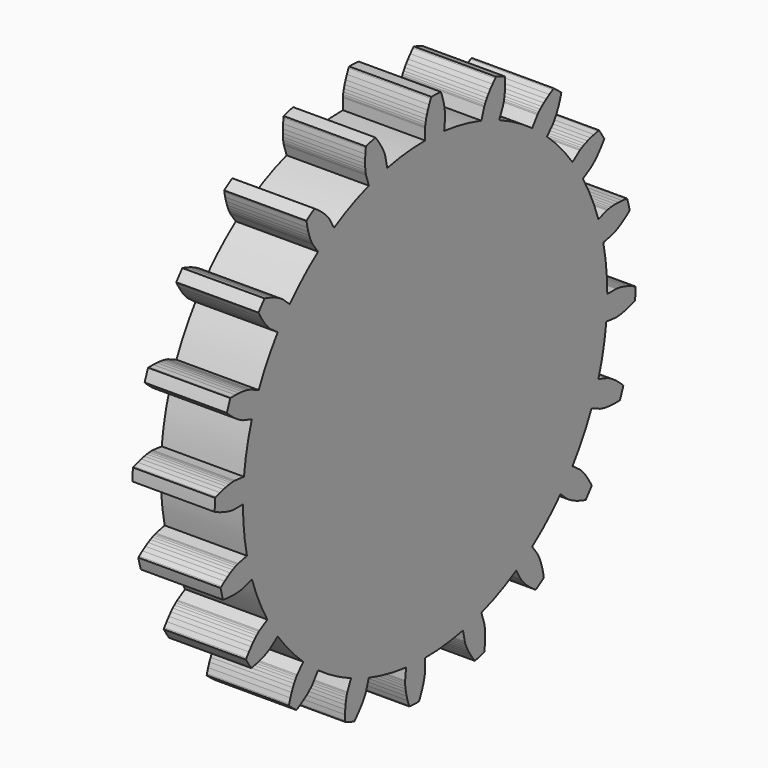
from build123d import *

# Parameters (mm, degrees)
F2_DEPTH = 12.7


# Not quite as in the source:
# - a variable given as a bare number and used for a length is read in inches; the dataset says mm whatever the document's units were


with BuildPart() as f2:
    # F1 (on Right) → F2 (new body)
    with BuildSketch(Plane.YZ):
        with BuildLine():
            ThreePointArc((34.9686031579, -3.6753482932), (35.11303277, -1.8401960714), (35.16122, 0))
            ThreePointArc((35.16122, 0), (34.9686031579, 3.6753482932), (34.3928629819, 7.3104287014))
            ThreePointArc((34.3928629819, 7.3104287014), (33.9631304818, 9.100393385), (33.4403074019, 10.865414523))
            ThreePointArc((33.4403074019, 10.865414523), (32.1213728162, 14.3013565892), (30.4505097481, 17.58061))
            ThreePointArc((30.4505097481, 17.58061), (29.4886803471, 19.1501729308), (28.446024523, 20.6672465686))
            ThreePointArc((28.446024523, 20.6672465686), (26.1298787005, 23.5274484589), (23.5274484589, 26.1298787005))
            ThreePointArc((23.5274484589, 26.1298787005), (22.1276727202, 27.3254001229), (20.6672465686, 28.446024523))
            ThreePointArc((20.6672465686, 28.446024523), (17.58061, 30.4505097481), (14.3013565892, 32.1213728162))
            ThreePointArc((14.3013565892, 32.1213728162), (12.6006543149, 32.8258267638), (10.865414523, 33.4403074019))
            ThreePointArc((10.865414523, 33.4403074019), (7.3104287014, 34.3928629819), (3.6753482932, 34.9686031579))
            ThreePointArc((3.6753482932, 34.9686031579), (1.8401960714, 35.11303277), (0, 35.16122))
            ThreePointArc((0, 35.16122), (-3.6753482932, 34.9686031579), (-7.3104287014, 34.3928629819))
            ThreePointArc((-7.3104287014, 34.3928629819), (-9.100393385, 33.9631304818), (-10.865414523, 33.4403074019))
            ThreePointArc((-10.865414523, 33.4403074019), (-14.3013565892, 32.1213728162), (-17.58061, 30.4505097481))
            ThreePointArc((-17.58061, 30.4505097481), (-19.1501729308, 29.4886803471), (-20.6672465686, 28.446024523))
            ThreePointArc((-20.6672465686, 28.446024523), (-23.5274484589, 26.1298787005), (-26.1298787005, 23.5274484589))
            ThreePointArc((-26.1298787005, 23.5274484589), (-27.3254001229, 22.1276727202), (-28.446024523, 20.6672465686))
            ThreePointArc((-28.446024523, 20.6672465686), (-30.4505097481, 17.58061), (-32.1213728162, 14.3013565892))
            ThreePointArc((-32.1213728162, 14.3013565892), (-32.8258267638, 12.6006543149), (-33.4403074019, 10.865414523))
            ThreePointArc((-33.4403074019, 10.865414523), (-34.3928629819, 7.3104287014), (-34.9686031579, 3.6753482932))
            ThreePointArc((-34.9686031579, 3.6753482932), (-35.11303277, 1.8401960714), (-35.16122, 0))
            ThreePointArc((-35.16122, 0), (-34.9686031579, -3.6753482932), (-34.3928629819, -7.3104287014))
            ThreePointArc((-34.3928629819, -7.3104287014), (-33.9631304818, -9.100393385), (-33.4403074019, -10.865414523))
            ThreePointArc((-33.4403074019, -10.865414523), (-32.1213728162, -14.3013565892), (-30.4505097481, -17.58061))
            ThreePointArc((-30.4505097481, -17.58061), (-29.4886803471, -19.1501729308), (-28.446024523, -20.6672465686))
            ThreePointArc((-28.446024523, -20.6672465686), (-26.1298787005, -23.5274484589), (-23.5274484589, -26.1298787005))
            ThreePointArc((-23.5274484589, -26.1298787005), (-22.1276727202, -27.3254001229), (-20.6672465686, -28.446024523))
            ThreePointArc((-20.6672465686, -28.446024523), (-17.58061, -30.4505097481), (-14.3013565892, -32.1213728162))
            ThreePointArc((-14.3013565892, -32.1213728162), (-12.6006543149, -32.8258267638), (-10.865414523, -33.4403074019))
            ThreePointArc((-10.865414523, -33.4403074019), (-7.3104287014, -34.3928629819), (-3.6753482932, -34.9686031579))
            ThreePointArc((-3.6753482932, -34.9686031579), (-1.8401960714, -35.11303277), (0, -35.16122))
            ThreePointArc((0, -35.16122), (3.6753482932, -34.9686031579), (7.3104287014, -34.3928629819))
            ThreePointArc((7.3104287014, -34.3928629819), (9.100393385, -33.9631304818), (10.865414523, -33.4403074019))
            ThreePointArc((10.865414523, -33.4403074019), (14.3013565892, -32.1213728162), (17.58061, -30.4505097481))
            ThreePointArc((17.58061, -30.4505097481), (19.1501729308, -29.4886803471), (20.6672465686, -28.446024523))
            ThreePointArc((20.6672465686, -28.446024523), (23.5274484589, -26.1298787005), (26.1298787005, -23.5274484589))
            ThreePointArc((26.1298787005, -23.5274484589), (27.3254001229, -22.1276727202), (28.446024523, -20.6672465686))
            ThreePointArc((28.446024523, -20.6672465686), (30.4505097481, -17.58061), (32.1213728162, -14.3013565892))
            ThreePointArc((32.1213728162, -14.3013565892), (32.8258267638, -12.6006543149), (33.4403074019, -10.865414523))
            ThreePointArc((33.4403074019, -10.865414523), (34.3928629819, -7.3104287014), (34.9686031579, -3.6753482932))
        make_face()
        with BuildLine():
            Line((-35.0810749527, -11.3985322171), (-33.4403074019, -10.865414523))
            ThreePointArc((-33.4403074019, -10.865414523), (-33.9631304818, -9.100393385), (-34.3928629819, -7.3104287014))
            Line((-34.3928629819, -7.3104287014), (-36.0803682097, -7.6691190104))
            Line((-36.0803682097, -7.6691190104), (-36.125121025, -7.6802023647))
            Line((-36.125121025, -7.6802023647), (-36.2577654905, -7.7193835081))
            Line((-36.2577654905, -7.7193835081), (-36.4753836489, -7.7954109725))
            Line((-36.4753836489, -7.7954109725), (-36.7744062464, -7.9168008706))
            Line((-36.7744062464, -7.9168008706), (-37.1506292157, -8.0917938492))
            Line((-37.1506292157, -8.0917938492), (-37.5992328238, -8.3283131361))
            Line((-37.5992328238, -8.3283131361), (-38.1148034149, -8.633923839))
            Line((-38.1148034149, -8.633923839), (-38.6913576712, -9.0157936503))
            Line((-38.6913576712, -9.0157936503), (-39.3223693016, -9.4806551065))
            Line((-39.3223693016, -9.4806551065), (-39.4863231421, -9.6145662784))
            ThreePointArc((-39.4863231421, -9.6145662784), (-39.2552255804, -10.518405993), (-39.0034420822, -11.4167029276))
            Line((-39.0034420822, -11.4167029276), (-38.7944983054, -11.450696484))
            Line((-38.7944983054, -11.450696484), (-38.0155954753, -11.5377724992))
            Line((-38.0155954753, -11.5377724992), (-37.3253499371, -11.5802043285))
            Line((-37.3253499371, -11.5802043285), (-36.7260473563, -11.5870856653))
            Line((-36.7260473563, -11.5870856653), (-36.219285592, -11.5676155722))
            Line((-36.219285592, -11.5676155722), (-35.8059704538, -11.5310524525))
            Line((-35.8059704538, -11.5310524525), (-35.486314339, -11.4866678893))
            Line((-35.486314339, -11.4866678893), (-35.2598377532, -11.4437005257))
            Line((-35.2598377532, -11.4437005257), (-35.1253737048, -11.4113101584))
            Line((-35.1253737048, -11.4113101584), (-35.0810749527, -11.3985322171))
        make_face()
        with BuildLine():
            Line((-29.8417447663, -21.6812966826), (-28.446024523, -20.6672465686))
            ThreePointArc((-28.446024523, -20.6672465686), (-29.4886803471, -19.1501729308), (-30.4505097481, -17.58061))
            Line((-30.4505097481, -17.58061), (-31.94458119, -18.4432125492))
            Line((-31.94458119, -18.4432125492), (-31.9837187018, -18.467582826))
            Line((-31.9837187018, -18.467582826), (-32.0977634459, -18.5458357018))
            Line((-32.0977634459, -18.5458357018), (-32.281236835, -18.6853898264))
            Line((-32.281236835, -18.6853898264), (-32.5281126834, -18.8932415444))
            Line((-32.5281126834, -18.8932415444), (-32.8318461857, -19.1759290482))
            Line((-32.8318461857, -19.1759290482), (-33.1854050912, -19.5394983959))
            Line((-33.1854050912, -19.5394983959), (-33.5813029607, -19.9894715208))
            Line((-33.5813029607, -19.9894715208), (-34.0116343818, -20.5308163565))
            Line((-34.0116343818, -20.5308163565), (-34.4681120147, -21.1679191911))
            Line((-34.4681120147, -21.1679191911), (-34.5826605552, -21.3459408067))
            ThreePointArc((-34.5826605552, -21.3459408067), (-34.0835718813, -22.134130383), (-33.5665225259, -22.9106561564))
            Line((-33.5665225259, -22.9106561564), (-33.3573005988, -22.8784187719))
            Line((-33.3573005988, -22.8784187719), (-32.5896120182, -22.7205387721))
            Line((-32.5896120182, -22.7205387721), (-31.9200373448, -22.5475962382))
            Line((-31.9200373448, -22.5475962382), (-31.3479402701, -22.3689460962))
            Line((-31.3479402701, -22.3689460962), (-30.8719977816, -22.19383094))
            Line((-30.8719977816, -22.19383094), (-30.4902103515, -22.031335945))
            Line((-30.4902103515, -22.031335945), (-30.1999149048, -21.8903445451))
            Line((-30.1999149048, -21.8903445451), (-29.9978005178, -21.7794950401))
            Line((-29.9978005178, -21.7794950401), (-29.8799267822, -21.7071382942))
            Line((-29.8799267822, -21.7071382942), (-29.8417447663, -21.6812966826))
        make_face()
        with BuildLine():
            Line((-21.6812966826, -29.8417447663), (-20.6672465686, -28.446024523))
            ThreePointArc((-20.6672465686, -28.446024523), (-22.1276727202, -27.3254001229), (-23.5274484589, -26.1298787005))
            Line((-23.5274484589, -26.1298787005), (-24.6818359925, -27.4119559422))
            Line((-24.6818359925, -27.4119559422), (-24.7115271484, -27.4472276091))
            Line((-24.7115271484, -27.4472276091), (-24.795808677, -27.5568922805))
            Line((-24.795808677, -27.5568922805), (-24.9271776431, -27.7463125354))
            Line((-24.9271776431, -27.7463125354), (-25.0977408143, -28.0202800989))
            Line((-25.0977408143, -28.0202800989), (-25.2992532981, -28.3829907054))
            Line((-25.2992532981, -28.3829907054), (-25.523158692, -28.8380214129))
            Line((-25.523158692, -28.8380214129), (-25.7606305979, -29.3883104552))
            Line((-25.7606305979, -29.3883104552), (-26.0026153461, -30.0361397112))
            Line((-26.0026153461, -30.0361397112), (-26.2398757704, -30.7831198597))
            Line((-26.2398757704, -30.7831198597), (-26.2938062017, -30.9878259229))
            ThreePointArc((-26.2938062017, -30.9878259229), (-25.5755806923, -31.5832118736), (-24.843877873, -32.1619547327))
            Line((-24.843877873, -32.1619547327), (-24.6548578956, -32.066642027))
            Line((-24.6548578956, -32.066642027), (-23.9735302715, -31.6792604066))
            Line((-23.9735302715, -31.6792604066), (-23.3901690973, -31.3078723298))
            Line((-23.3901690973, -31.3078723298), (-22.9012783763, -30.9611782295))
            Line((-22.9012783763, -30.9611782295), (-22.5027437305, -30.6475595019))
            Line((-22.5027437305, -30.6475595019), (-22.1898560222, -30.3750387739))
            Line((-22.1898560222, -30.3750387739), (-21.9573373846, -30.1512417578))
            Line((-21.9573373846, -30.1512417578), (-21.7993695606, -29.9833608334))
            Line((-21.7993695606, -29.9833608334), (-21.7096244405, -29.8781204912))
            Line((-21.7096244405, -29.8781204912), (-21.6812966826, -29.8417447663))
        make_face()
        with BuildLine():
            Line((-11.3985322171, -35.0810749527), (-10.865414523, -33.4403074019))
            ThreePointArc((-10.865414523, -33.4403074019), (-12.6006543149, -32.8258267638), (-14.3013565892, -32.1213728162))
            Line((-14.3013565892, -32.1213728162), (-15.0030607196, -33.6974260973))
            Line((-15.0030607196, -33.6974260973), (-15.0203991425, -33.7401465177))
            Line((-15.0203991425, -33.7401465177), (-15.0666673922, -33.8704882427))
            Line((-15.0666673922, -33.8704882427), (-15.1330726256, -34.0912328535))
            Line((-15.1330726256, -34.0912328535), (-15.210627208, -34.4044984085))
            Line((-15.210627208, -34.4044984085), (-15.2901932274, -34.8117274764))
            Line((-15.2901932274, -34.8117274764), (-15.3625276897, -35.3136779678))
            Line((-15.3625276897, -35.3136779678), (-15.4183282274, -35.9104168019))
            Line((-15.4183282274, -35.9104168019), (-15.4482791495, -36.6013164368))
            Line((-15.4482791495, -36.6013164368), (-15.4430976617, -37.3850542778))
            Line((-15.4430976617, -37.3850542778), (-15.4311308974, -37.5964067329))
            ThreePointArc((-15.4311308974, -37.5964067329), (-14.5640734695, -37.9407085328), (-13.6893413564, -38.2650170943))
            Line((-13.6893413564, -38.2650170943), (-13.539025921, -38.1159589391))
            Line((-13.539025921, -38.1159589391), (-13.0107523484, -37.5369953102))
            Line((-13.0107523484, -37.5369953102), (-12.5707081296, -37.0035157429))
            Line((-12.5707081296, -37.0035157429), (-12.2128797925, -36.5227145185))
            Line((-12.2128797925, -36.5227145185), (-11.9307643372, -36.1012914056))
            Line((-11.9307643372, -36.1012914056), (-11.7174039796, -35.7454211722))
            Line((-11.7174039796, -35.7454211722), (-11.5654226955, -35.4607253513))
            Line((-11.5654226955, -35.4607253513), (-11.4670644258, -35.2522463619))
            Line((-11.4670644258, -35.2522463619), (-11.4142327987, -35.1244240814))
            Line((-11.4142327987, -35.1244240814), (-11.3985322171, -35.0810749527))
        make_face()
        with BuildLine():
            Line((0, -36.8864250984), (0, -35.16122))
            ThreePointArc((0, -35.16122), (-1.8401960714, -35.11303277), (-3.6753482932, -34.9686031579))
            Line((-3.6753482932, -34.9686031579), (-3.855681331, -36.6843574022))
            Line((-3.855681331, -36.6843574022), (-3.8589698151, -36.7303448037))
            Line((-3.8589698151, -36.7303448037), (-3.8626957275, -36.8686048261))
            Line((-3.8626957275, -36.8686048261), (-3.8576370213, -37.0990657723))
            Line((-3.8576370213, -37.0990657723), (-3.834591432, -37.4209647036))
            Line((-3.834591432, -37.4209647036), (-3.7844225105, -37.8328498145))
            Line((-3.7844225105, -37.8328498145), (-3.6981054401, -38.3325856783))
            Line((-3.6981054401, -38.3325856783), (-3.5667724642, -38.9173613495))
            Line((-3.5667724642, -38.9173613495), (-3.3817577552, -39.5837012932))
            Line((-3.3817577552, -39.5837012932), (-3.1346415555, -40.3274791062))
            Line((-3.1346415555, -40.3274791062), (-3.0579489859, -40.5247893023))
            ThreePointArc((-3.0579489859, -40.5247893023), (-2.1269332617, -40.5843042924), (-1.1947967286, -40.6224329746))
            Line((-1.1947967286, -40.6224329746), (-1.0978997574, -40.4342202208))
            Line((-1.0978997574, -40.4342202208), (-0.7743913343, -39.7203475771))
            Line((-0.7743913343, -39.7203475771), (-0.5207386649, -39.0769972165))
            Line((-0.5207386649, -39.0769972165), (-0.3289994424, -38.5091530418))
            Line((-0.3289994424, -38.5091530418), (-0.1909186041, -38.0211773741))
            Line((-0.1909186041, -38.0211773741), (-0.0979707956, -37.6167926932))
            Line((-0.0979707956, -37.6167926932), (-0.0414038518, -37.2990660779))
            Line((-0.0414038518, -37.2990660779), (-0.0122831292, -37.0703963997))
            Line((-0.0122831292, -37.0703963997), (-0.0015365229, -36.9325043163))
            Line((-0.0015365229, -36.9325043163), (0, -36.8864250984))
        make_face()
        with BuildLine():
            Line((11.3985322171, -35.0810749527), (10.865414523, -33.4403074019))
            ThreePointArc((10.865414523, -33.4403074019), (9.100393385, -33.9631304818), (7.3104287014, -34.3928629819))
            Line((7.3104287014, -34.3928629819), (7.6691190104, -36.0803682097))
            Line((7.6691190104, -36.0803682097), (7.6802023647, -36.125121025))
            Line((7.6802023647, -36.125121025), (7.7193835081, -36.2577654905))
            Line((7.7193835081, -36.2577654905), (7.7954109725, -36.4753836489))
            Line((7.7954109725, -36.4753836489), (7.9168008706, -36.7744062464))
            Line((7.9168008706, -36.7744062464), (8.0917938492, -37.1506292157))
            Line((8.0917938492, -37.1506292157), (8.3283131361, -37.5992328238))
            Line((8.3283131361, -37.5992328238), (8.633923839, -38.1148034149))
            Line((8.633923839, -38.1148034149), (9.0157936503, -38.6913576712))
            Line((9.0157936503, -38.6913576712), (9.4806551065, -39.3223693016))
            Line((9.4806551065, -39.3223693016), (9.6145662784, -39.4863231421))
            ThreePointArc((9.6145662784, -39.4863231421), (10.518405993, -39.2552255804), (11.4167029276, -39.0034420822))
            Line((11.4167029276, -39.0034420822), (11.450696484, -38.7944983054))
            Line((11.450696484, -38.7944983054), (11.5377724992, -38.0155954753))
            Line((11.5377724992, -38.0155954753), (11.5802043285, -37.3253499371))
            Line((11.5802043285, -37.3253499371), (11.5870856653, -36.7260473563))
            Line((11.5870856653, -36.7260473563), (11.5676155722, -36.219285592))
            Line((11.5676155722, -36.219285592), (11.5310524525, -35.8059704538))
            Line((11.5310524525, -35.8059704538), (11.4866678893, -35.486314339))
            Line((11.4866678893, -35.486314339), (11.4437005257, -35.2598377532))
            Line((11.4437005257, -35.2598377532), (11.4113101584, -35.1253737048))
            Line((11.4113101584, -35.1253737048), (11.3985322171, -35.0810749527))
        make_face()
        with BuildLine():
            Line((21.6812966826, -29.8417447663), (20.6672465686, -28.446024523))
            ThreePointArc((20.6672465686, -28.446024523), (19.1501729308, -29.4886803471), (17.58061, -30.4505097481))
            Line((17.58061, -30.4505097481), (18.4432125492, -31.94458119))
            Line((18.4432125492, -31.94458119), (18.467582826, -31.9837187018))
            Line((18.467582826, -31.9837187018), (18.5458357018, -32.0977634459))
            Line((18.5458357018, -32.0977634459), (18.6853898264, -32.281236835))
            Line((18.6853898264, -32.281236835), (18.8932415444, -32.5281126834))
            Line((18.8932415444, -32.5281126834), (19.1759290482, -32.8318461857))
            Line((19.1759290482, -32.8318461857), (19.5394983959, -33.1854050912))
            Line((19.5394983959, -33.1854050912), (19.9894715208, -33.5813029607))
            Line((19.9894715208, -33.5813029607), (20.5308163565, -34.0116343818))
            Line((20.5308163565, -34.0116343818), (21.1679191911, -34.4681120147))
            Line((21.1679191911, -34.4681120147), (21.3459408067, -34.5826605552))
            ThreePointArc((21.3459408067, -34.5826605552), (22.134130383, -34.0835718813), (22.9106561564, -33.5665225259))
            Line((22.9106561564, -33.5665225259), (22.8784187719, -33.3573005988))
            Line((22.8784187719, -33.3573005988), (22.7205387721, -32.5896120182))
            Line((22.7205387721, -32.5896120182), (22.5475962382, -31.9200373448))
            Line((22.5475962382, -31.9200373448), (22.3689460962, -31.3479402701))
            Line((22.3689460962, -31.3479402701), (22.19383094, -30.8719977816))
            Line((22.19383094, -30.8719977816), (22.031335945, -30.4902103515))
            Line((22.031335945, -30.4902103515), (21.8903445451, -30.1999149048))
            Line((21.8903445451, -30.1999149048), (21.7794950401, -29.9978005178))
            Line((21.7794950401, -29.9978005178), (21.7071382942, -29.8799267822))
            Line((21.7071382942, -29.8799267822), (21.6812966826, -29.8417447663))
        make_face()
        with BuildLine():
            Line((29.8417447663, -21.6812966826), (28.446024523, -20.6672465686))
            ThreePointArc((28.446024523, -20.6672465686), (27.3254001229, -22.1276727202), (26.1298787005, -23.5274484589))
            Line((26.1298787005, -23.5274484589), (27.4119559422, -24.6818359925))
            Line((27.4119559422, -24.6818359925), (27.4472276091, -24.7115271484))
            Line((27.4472276091, -24.7115271484), (27.5568922805, -24.795808677))
            Line((27.5568922805, -24.795808677), (27.7463125354, -24.9271776431))
            Line((27.7463125354, -24.9271776431), (28.0202800989, -25.0977408143))
            Line((28.0202800989, -25.0977408143), (28.3829907054, -25.2992532981))
            Line((28.3829907054, -25.2992532981), (28.8380214129, -25.523158692))
            Line((28.8380214129, -25.523158692), (29.3883104552, -25.7606305979))
            Line((29.3883104552, -25.7606305979), (30.0361397112, -26.0026153461))
            Line((30.0361397112, -26.0026153461), (30.7831198597, -26.2398757704))
            Line((30.7831198597, -26.2398757704), (30.9878259229, -26.2938062017))
            ThreePointArc((30.9878259229, -26.2938062017), (31.5832118736, -25.5755806923), (32.1619547327, -24.843877873))
            Line((32.1619547327, -24.843877873), (32.066642027, -24.6548578956))
            Line((32.066642027, -24.6548578956), (31.6792604066, -23.9735302715))
            Line((31.6792604066, -23.9735302715), (31.3078723298, -23.3901690973))
            Line((31.3078723298, -23.3901690973), (30.9611782295, -22.9012783763))
            Line((30.9611782295, -22.9012783763), (30.6475595019, -22.5027437305))
            Line((30.6475595019, -22.5027437305), (30.3750387739, -22.1898560222))
            Line((30.3750387739, -22.1898560222), (30.1512417578, -21.9573373846))
            Line((30.1512417578, -21.9573373846), (29.9833608334, -21.7993695606))
            Line((29.9833608334, -21.7993695606), (29.8781204912, -21.7096244405))
            Line((29.8781204912, -21.7096244405), (29.8417447663, -21.6812966826))
        make_face()
        with BuildLine():
            Line((35.0810749527, -11.3985322171), (33.4403074019, -10.865414523))
            ThreePointArc((33.4403074019, -10.865414523), (32.8258267638, -12.6006543149), (32.1213728162, -14.3013565892))
            Line((32.1213728162, -14.3013565892), (33.6974260973, -15.0030607196))
            Line((33.6974260973, -15.0030607196), (33.7401465177, -15.0203991425))
            Line((33.7401465177, -15.0203991425), (33.8704882427, -15.0666673922))
            Line((33.8704882427, -15.0666673922), (34.0912328535, -15.1330726256))
            Line((34.0912328535, -15.1330726256), (34.4044984085, -15.210627208))
            Line((34.4044984085, -15.210627208), (34.8117274764, -15.2901932274))
            Line((34.8117274764, -15.2901932274), (35.3136779678, -15.3625276897))
            Line((35.3136779678, -15.3625276897), (35.9104168019, -15.4183282274))
            Line((35.9104168019, -15.4183282274), (36.6013164368, -15.4482791495))
            Line((36.6013164368, -15.4482791495), (37.3850542778, -15.4430976617))
            Line((37.3850542778, -15.4430976617), (37.5964067329, -15.4311308974))
            ThreePointArc((37.5964067329, -15.4311308974), (37.9407085328, -14.5640734695), (38.2650170943, -13.6893413564))
            Line((38.2650170943, -13.6893413564), (38.1159589391, -13.539025921))
            Line((38.1159589391, -13.539025921), (37.5369953102, -13.0107523484))
            Line((37.5369953102, -13.0107523484), (37.0035157429, -12.5707081296))
            Line((37.0035157429, -12.5707081296), (36.5227145185, -12.2128797925))
            Line((36.5227145185, -12.2128797925), (36.1012914056, -11.9307643372))
            Line((36.1012914056, -11.9307643372), (35.7454211722, -11.7174039796))
            Line((35.7454211722, -11.7174039796), (35.4607253513, -11.5654226955))
            Line((35.4607253513, -11.5654226955), (35.2522463619, -11.4670644258))
            Line((35.2522463619, -11.4670644258), (35.1244240814, -11.4142327987))
            Line((35.1244240814, -11.4142327987), (35.0810749527, -11.3985322171))
        make_face()
        with BuildLine():
            Line((36.8864250984, 0), (35.16122, 0))
            ThreePointArc((35.16122, 0), (35.11303277, -1.8401960714), (34.9686031579, -3.6753482932))
            Line((34.9686031579, -3.6753482932), (36.6843574022, -3.855681331))
            Line((36.6843574022, -3.855681331), (36.7303448037, -3.8589698151))
            Line((36.7303448037, -3.8589698151), (36.8686048261, -3.8626957275))
            Line((36.8686048261, -3.8626957275), (37.0990657723, -3.8576370213))
            Line((37.0990657723, -3.8576370213), (37.4209647036, -3.834591432))
            Line((37.4209647036, -3.834591432), (37.8328498145, -3.7844225105))
            Line((37.8328498145, -3.7844225105), (38.3325856783, -3.6981054401))
            Line((38.3325856783, -3.6981054401), (38.9173613495, -3.5667724642))
            Line((38.9173613495, -3.5667724642), (39.5837012932, -3.3817577552))
            Line((39.5837012932, -3.3817577552), (40.3274791062, -3.1346415555))
            Line((40.3274791062, -3.1346415555), (40.5247893023, -3.0579489859))
            ThreePointArc((40.5247893023, -3.0579489859), (40.5843042924, -2.1269332617), (40.6224329746, -1.1947967286))
            Line((40.6224329746, -1.1947967286), (40.4342202208, -1.0978997574))
            Line((40.4342202208, -1.0978997574), (39.7203475771, -0.7743913343))
            Line((39.7203475771, -0.7743913343), (39.0769972165, -0.5207386649))
            Line((39.0769972165, -0.5207386649), (38.5091530418, -0.3289994424))
            Line((38.5091530418, -0.3289994424), (38.0211773741, -0.1909186041))
            Line((38.0211773741, -0.1909186041), (37.6167926932, -0.0979707956))
            Line((37.6167926932, -0.0979707956), (37.2990660779, -0.0414038518))
            Line((37.2990660779, -0.0414038518), (37.0703963997, -0.0122831292))
            Line((37.0703963997, -0.0122831292), (36.9325043163, -0.0015365229))
            Line((36.9325043163, -0.0015365229), (36.8864250984, 0))
        make_face()
        with BuildLine():
            ThreePointArc((33.4403074019, 10.865414523), (33.9631304818, 9.100393385), (34.3928629819, 7.3104287014))
            Line((34.3928629819, 7.3104287014), (36.0803682097, 7.6691190104))
            Line((36.0803682097, 7.6691190104), (36.125121025, 7.6802023647))
            Line((36.125121025, 7.6802023647), (36.2577654905, 7.7193835081))
            Line((36.2577654905, 7.7193835081), (36.4753836489, 7.7954109725))
            Line((36.4753836489, 7.7954109725), (36.7744062464, 7.9168008706))
            Line((36.7744062464, 7.9168008706), (37.1506292157, 8.0917938492))
            Line((37.1506292157, 8.0917938492), (37.5992328238, 8.3283131361))
            Line((37.5992328238, 8.3283131361), (38.1148034149, 8.633923839))
            Line((38.1148034149, 8.633923839), (38.6913576712, 9.0157936503))
            Line((38.6913576712, 9.0157936503), (39.3223693016, 9.4806551065))
            Line((39.3223693016, 9.4806551065), (39.4863231421, 9.6145662784))
            ThreePointArc((39.4863231421, 9.6145662784), (39.2552255804, 10.518405993), (39.0034420822, 11.4167029276))
            Line((39.0034420822, 11.4167029276), (38.7944983054, 11.450696484))
            Line((38.7944983054, 11.450696484), (38.0155954753, 11.5377724992))
            Line((38.0155954753, 11.5377724992), (37.3253499371, 11.5802043285))
            Line((37.3253499371, 11.5802043285), (36.7260473563, 11.5870856653))
            Line((36.7260473563, 11.5870856653), (36.219285592, 11.5676155722))
            Line((36.219285592, 11.5676155722), (35.8059704538, 11.5310524525))
            Line((35.8059704538, 11.5310524525), (35.486314339, 11.4866678893))
            Line((35.486314339, 11.4866678893), (35.2598377532, 11.4437005257))
            Line((35.2598377532, 11.4437005257), (35.1253737048, 11.4113101584))
            Line((35.1253737048, 11.4113101584), (35.0810749527, 11.3985322171))
            Line((35.0810749527, 11.3985322171), (33.4403074019, 10.865414523))
        make_face()
        with BuildLine():
            ThreePointArc((28.446024523, 20.6672465686), (29.4886803471, 19.1501729308), (30.4505097481, 17.58061))
            Line((30.4505097481, 17.58061), (31.94458119, 18.4432125492))
            Line((31.94458119, 18.4432125492), (31.9837187018, 18.467582826))
            Line((31.9837187018, 18.467582826), (32.0977634459, 18.5458357018))
            Line((32.0977634459, 18.5458357018), (32.281236835, 18.6853898264))
            Line((32.281236835, 18.6853898264), (32.5281126834, 18.8932415444))
            Line((32.5281126834, 18.8932415444), (32.8318461857, 19.1759290482))
            Line((32.8318461857, 19.1759290482), (33.1854050912, 19.5394983959))
            Line((33.1854050912, 19.5394983959), (33.5813029607, 19.9894715208))
            Line((33.5813029607, 19.9894715208), (34.0116343818, 20.5308163565))
            Line((34.0116343818, 20.5308163565), (34.4681120147, 21.1679191911))
            Line((34.4681120147, 21.1679191911), (34.5826605552, 21.3459408067))
            ThreePointArc((34.5826605552, 21.3459408067), (34.0835718813, 22.134130383), (33.5665225259, 22.9106561564))
            Line((33.5665225259, 22.9106561564), (33.3573005988, 22.8784187719))
            Line((33.3573005988, 22.8784187719), (32.5896120182, 22.7205387721))
            Line((32.5896120182, 22.7205387721), (31.9200373448, 22.5475962382))
            Line((31.9200373448, 22.5475962382), (31.3479402701, 22.3689460962))
            Line((31.3479402701, 22.3689460962), (30.8719977816, 22.19383094))
            Line((30.8719977816, 22.19383094), (30.4902103515, 22.031335945))
            Line((30.4902103515, 22.031335945), (30.1999149048, 21.8903445451))
            Line((30.1999149048, 21.8903445451), (29.9978005178, 21.7794950401))
            Line((29.9978005178, 21.7794950401), (29.8799267822, 21.7071382942))
            Line((29.8799267822, 21.7071382942), (29.8417447663, 21.6812966826))
            Line((29.8417447663, 21.6812966826), (28.446024523, 20.6672465686))
        make_face()
        with BuildLine():
            ThreePointArc((20.6672465686, 28.446024523), (22.1276727202, 27.3254001229), (23.5274484589, 26.1298787005))
            Line((23.5274484589, 26.1298787005), (24.6818359925, 27.4119559422))
            Line((24.6818359925, 27.4119559422), (24.7115271484, 27.4472276091))
            Line((24.7115271484, 27.4472276091), (24.795808677, 27.5568922805))
            Line((24.795808677, 27.5568922805), (24.9271776431, 27.7463125354))
            Line((24.9271776431, 27.7463125354), (25.0977408143, 28.0202800989))
            Line((25.0977408143, 28.0202800989), (25.2992532981, 28.3829907054))
            Line((25.2992532981, 28.3829907054), (25.523158692, 28.8380214129))
            Line((25.523158692, 28.8380214129), (25.7606305979, 29.3883104552))
            Line((25.7606305979, 29.3883104552), (26.0026153461, 30.0361397112))
            Line((26.0026153461, 30.0361397112), (26.2398757704, 30.7831198597))
            Line((26.2398757704, 30.7831198597), (26.2938062017, 30.9878259229))
            ThreePointArc((26.2938062017, 30.9878259229), (25.5755806923, 31.5832118736), (24.843877873, 32.1619547327))
            Line((24.843877873, 32.1619547327), (24.6548578956, 32.066642027))
            Line((24.6548578956, 32.066642027), (23.9735302715, 31.6792604066))
            Line((23.9735302715, 31.6792604066), (23.3901690973, 31.3078723298))
            Line((23.3901690973, 31.3078723298), (22.9012783763, 30.9611782295))
            Line((22.9012783763, 30.9611782295), (22.5027437305, 30.6475595019))
            Line((22.5027437305, 30.6475595019), (22.1898560222, 30.3750387739))
            Line((22.1898560222, 30.3750387739), (21.9573373846, 30.1512417578))
            Line((21.9573373846, 30.1512417578), (21.7993695606, 29.9833608334))
            Line((21.7993695606, 29.9833608334), (21.7096244405, 29.8781204912))
            Line((21.7096244405, 29.8781204912), (21.6812966826, 29.8417447663))
            Line((21.6812966826, 29.8417447663), (20.6672465686, 28.446024523))
        make_face()
        with BuildLine():
            ThreePointArc((10.865414523, 33.4403074019), (12.6006543149, 32.8258267638), (14.3013565892, 32.1213728162))
            Line((14.3013565892, 32.1213728162), (15.0030607196, 33.6974260973))
            Line((15.0030607196, 33.6974260973), (15.0203991425, 33.7401465177))
            Line((15.0203991425, 33.7401465177), (15.0666673922, 33.8704882427))
            Line((15.0666673922, 33.8704882427), (15.1330726256, 34.0912328535))
            Line((15.1330726256, 34.0912328535), (15.210627208, 34.4044984085))
            Line((15.210627208, 34.4044984085), (15.2901932274, 34.8117274764))
            Line((15.2901932274, 34.8117274764), (15.3625276897, 35.3136779678))
            Line((15.3625276897, 35.3136779678), (15.4183282274, 35.9104168019))
            Line((15.4183282274, 35.9104168019), (15.4482791495, 36.6013164368))
            Line((15.4482791495, 36.6013164368), (15.4430976617, 37.3850542778))
            Line((15.4430976617, 37.3850542778), (15.4311308974, 37.5964067329))
            ThreePointArc((15.4311308974, 37.5964067329), (14.5640734695, 37.9407085328), (13.6893413564, 38.2650170943))
            Line((13.6893413564, 38.2650170943), (13.539025921, 38.1159589391))
            Line((13.539025921, 38.1159589391), (13.0107523484, 37.5369953102))
            Line((13.0107523484, 37.5369953102), (12.5707081296, 37.0035157429))
            Line((12.5707081296, 37.0035157429), (12.2128797925, 36.5227145185))
            Line((12.2128797925, 36.5227145185), (11.9307643372, 36.1012914056))
            Line((11.9307643372, 36.1012914056), (11.7174039796, 35.7454211722))
            Line((11.7174039796, 35.7454211722), (11.5654226955, 35.4607253513))
            Line((11.5654226955, 35.4607253513), (11.4670644258, 35.2522463619))
            Line((11.4670644258, 35.2522463619), (11.4142327987, 35.1244240814))
            Line((11.4142327987, 35.1244240814), (11.3985322171, 35.0810749527))
            Line((11.3985322171, 35.0810749527), (10.865414523, 33.4403074019))
        make_face()
        with BuildLine():
            ThreePointArc((0, 35.16122), (1.8401960714, 35.11303277), (3.6753482932, 34.9686031579))
            Line((3.6753482932, 34.9686031579), (3.855681331, 36.6843574022))
            Line((3.855681331, 36.6843574022), (3.8589698151, 36.7303448037))
            Line((3.8589698151, 36.7303448037), (3.8626957275, 36.8686048261))
            Line((3.8626957275, 36.8686048261), (3.8576370213, 37.0990657723))
            Line((3.8576370213, 37.0990657723), (3.834591432, 37.4209647036))
            Line((3.834591432, 37.4209647036), (3.7844225105, 37.8328498145))
            Line((3.7844225105, 37.8328498145), (3.6981054401, 38.3325856783))
            Line((3.6981054401, 38.3325856783), (3.5667724642, 38.9173613495))
            Line((3.5667724642, 38.9173613495), (3.3817577552, 39.5837012932))
            Line((3.3817577552, 39.5837012932), (3.1346415555, 40.3274791062))
            Line((3.1346415555, 40.3274791062), (3.0579489859, 40.5247893023))
            ThreePointArc((3.0579489859, 40.5247893023), (2.1269332617, 40.5843042924), (1.1947967286, 40.6224329746))
            Line((1.1947967286, 40.6224329746), (1.0978997574, 40.4342202208))
            Line((1.0978997574, 40.4342202208), (0.7743913343, 39.7203475771))
            Line((0.7743913343, 39.7203475771), (0.5207386649, 39.0769972165))
            Line((0.5207386649, 39.0769972165), (0.3289994424, 38.5091530418))
            Line((0.3289994424, 38.5091530418), (0.1909186041, 38.0211773741))
            Line((0.1909186041, 38.0211773741), (0.0979707956, 37.6167926932))
            Line((0.0979707956, 37.6167926932), (0.0414038518, 37.2990660779))
            Line((0.0414038518, 37.2990660779), (0.0122831292, 37.0703963997))
            Line((0.0122831292, 37.0703963997), (0.0015365229, 36.9325043163))
            Line((0.0015365229, 36.9325043163), (0, 36.8864250984))
            Line((0, 36.8864250984), (0, 35.16122))
        make_face()
        with BuildLine():
            ThreePointArc((-10.865414523, 33.4403074019), (-9.100393385, 33.9631304818), (-7.3104287014, 34.3928629819))
            Line((-7.3104287014, 34.3928629819), (-7.6691190104, 36.0803682097))
            Line((-7.6691190104, 36.0803682097), (-7.6802023647, 36.125121025))
            Line((-7.6802023647, 36.125121025), (-7.7193835081, 36.2577654905))
            Line((-7.7193835081, 36.2577654905), (-7.7954109725, 36.4753836489))
            Line((-7.7954109725, 36.4753836489), (-7.9168008706, 36.7744062464))
            Line((-7.9168008706, 36.7744062464), (-8.0917938492, 37.1506292157))
            Line((-8.0917938492, 37.1506292157), (-8.3283131361, 37.5992328238))
            Line((-8.3283131361, 37.5992328238), (-8.633923839, 38.1148034149))
            Line((-8.633923839, 38.1148034149), (-9.0157936503, 38.6913576712))
            Line((-9.0157936503, 38.6913576712), (-9.4806551065, 39.3223693016))
            Line((-9.4806551065, 39.3223693016), (-9.6145662784, 39.4863231421))
            ThreePointArc((-9.6145662784, 39.4863231421), (-10.518405993, 39.2552255804), (-11.4167029276, 39.0034420822))
            Line((-11.4167029276, 39.0034420822), (-11.450696484, 38.7944983054))
            Line((-11.450696484, 38.7944983054), (-11.5377724992, 38.0155954753))
            Line((-11.5377724992, 38.0155954753), (-11.5802043285, 37.3253499371))
            Line((-11.5802043285, 37.3253499371), (-11.5870856653, 36.7260473563))
            Line((-11.5870856653, 36.7260473563), (-11.5676155722, 36.219285592))
            Line((-11.5676155722, 36.219285592), (-11.5310524525, 35.8059704538))
            Line((-11.5310524525, 35.8059704538), (-11.4866678893, 35.486314339))
            Line((-11.4866678893, 35.486314339), (-11.4437005257, 35.2598377532))
            Line((-11.4437005257, 35.2598377532), (-11.4113101584, 35.1253737048))
            Line((-11.4113101584, 35.1253737048), (-11.3985322171, 35.0810749527))
            Line((-11.3985322171, 35.0810749527), (-10.865414523, 33.4403074019))
        make_face()
        with BuildLine():
            ThreePointArc((-20.6672465686, 28.446024523), (-19.1501729308, 29.4886803471), (-17.58061, 30.4505097481))
            Line((-17.58061, 30.4505097481), (-18.4432125492, 31.94458119))
            Line((-18.4432125492, 31.94458119), (-18.467582826, 31.9837187018))
            Line((-18.467582826, 31.9837187018), (-18.5458357018, 32.0977634459))
            Line((-18.5458357018, 32.0977634459), (-18.6853898264, 32.281236835))
            Line((-18.6853898264, 32.281236835), (-18.8932415444, 32.5281126834))
            Line((-18.8932415444, 32.5281126834), (-19.1759290482, 32.8318461857))
            Line((-19.1759290482, 32.8318461857), (-19.5394983959, 33.1854050912))
            Line((-19.5394983959, 33.1854050912), (-19.9894715208, 33.5813029607))
            Line((-19.9894715208, 33.5813029607), (-20.5308163565, 34.0116343818))
            Line((-20.5308163565, 34.0116343818), (-21.1679191911, 34.4681120147))
            Line((-21.1679191911, 34.4681120147), (-21.3459408067, 34.5826605552))
            ThreePointArc((-21.3459408067, 34.5826605552), (-22.134130383, 34.0835718813), (-22.9106561564, 33.5665225259))
            Line((-22.9106561564, 33.5665225259), (-22.8784187719, 33.3573005988))
            Line((-22.8784187719, 33.3573005988), (-22.7205387721, 32.5896120182))
            Line((-22.7205387721, 32.5896120182), (-22.5475962382, 31.9200373448))
            Line((-22.5475962382, 31.9200373448), (-22.3689460962, 31.3479402701))
            Line((-22.3689460962, 31.3479402701), (-22.19383094, 30.8719977816))
            Line((-22.19383094, 30.8719977816), (-22.031335945, 30.4902103515))
            Line((-22.031335945, 30.4902103515), (-21.8903445451, 30.1999149048))
            Line((-21.8903445451, 30.1999149048), (-21.7794950401, 29.9978005178))
            Line((-21.7794950401, 29.9978005178), (-21.7071382942, 29.8799267822))
            Line((-21.7071382942, 29.8799267822), (-21.6812966826, 29.8417447663))
            Line((-21.6812966826, 29.8417447663), (-20.6672465686, 28.446024523))
        make_face()
        with BuildLine():
            ThreePointArc((-28.446024523, 20.6672465686), (-27.3254001229, 22.1276727202), (-26.1298787005, 23.5274484589))
            Line((-26.1298787005, 23.5274484589), (-27.4119559422, 24.6818359925))
            Line((-27.4119559422, 24.6818359925), (-27.4472276091, 24.7115271484))
            Line((-27.4472276091, 24.7115271484), (-27.5568922805, 24.795808677))
            Line((-27.5568922805, 24.795808677), (-27.7463125354, 24.9271776431))
            Line((-27.7463125354, 24.9271776431), (-28.0202800989, 25.0977408143))
            Line((-28.0202800989, 25.0977408143), (-28.3829907054, 25.2992532981))
            Line((-28.3829907054, 25.2992532981), (-28.8380214129, 25.523158692))
            Line((-28.8380214129, 25.523158692), (-29.3883104552, 25.7606305979))
            Line((-29.3883104552, 25.7606305979), (-30.0361397112, 26.0026153461))
            Line((-30.0361397112, 26.0026153461), (-30.7831198597, 26.2398757704))
            Line((-30.7831198597, 26.2398757704), (-30.9878259229, 26.2938062017))
            ThreePointArc((-30.9878259229, 26.2938062017), (-31.5832118736, 25.5755806923), (-32.1619547327, 24.843877873))
            Line((-32.1619547327, 24.843877873), (-32.066642027, 24.6548578956))
            Line((-32.066642027, 24.6548578956), (-31.6792604066, 23.9735302715))
            Line((-31.6792604066, 23.9735302715), (-31.3078723298, 23.3901690973))
            Line((-31.3078723298, 23.3901690973), (-30.9611782295, 22.9012783763))
            Line((-30.9611782295, 22.9012783763), (-30.6475595019, 22.5027437305))
            Line((-30.6475595019, 22.5027437305), (-30.3750387739, 22.1898560222))
            Line((-30.3750387739, 22.1898560222), (-30.1512417578, 21.9573373846))
            Line((-30.1512417578, 21.9573373846), (-29.9833608334, 21.7993695606))
            Line((-29.9833608334, 21.7993695606), (-29.8781204912, 21.7096244405))
            Line((-29.8781204912, 21.7096244405), (-29.8417447663, 21.6812966826))
            Line((-29.8417447663, 21.6812966826), (-28.446024523, 20.6672465686))
        make_face()
        with BuildLine():
            ThreePointArc((-33.4403074019, 10.865414523), (-32.8258267638, 12.6006543149), (-32.1213728162, 14.3013565892))
            Line((-32.1213728162, 14.3013565892), (-33.6974260973, 15.0030607196))
            Line((-33.6974260973, 15.0030607196), (-33.7401465177, 15.0203991425))
            Line((-33.7401465177, 15.0203991425), (-33.8704882427, 15.0666673922))
            Line((-33.8704882427, 15.0666673922), (-34.0912328535, 15.1330726256))
            Line((-34.0912328535, 15.1330726256), (-34.4044984085, 15.210627208))
            Line((-34.4044984085, 15.210627208), (-34.8117274764, 15.2901932274))
            Line((-34.8117274764, 15.2901932274), (-35.3136779678, 15.3625276897))
            Line((-35.3136779678, 15.3625276897), (-35.9104168019, 15.4183282274))
            Line((-35.9104168019, 15.4183282274), (-36.6013164368, 15.4482791495))
            Line((-36.6013164368, 15.4482791495), (-37.3850542778, 15.4430976617))
            Line((-37.3850542778, 15.4430976617), (-37.5964067329, 15.4311308974))
            ThreePointArc((-37.5964067329, 15.4311308974), (-37.9407085328, 14.5640734695), (-38.2650170943, 13.6893413564))
            Line((-38.2650170943, 13.6893413564), (-38.1159589391, 13.539025921))
            Line((-38.1159589391, 13.539025921), (-37.5369953102, 13.0107523484))
            Line((-37.5369953102, 13.0107523484), (-37.0035157429, 12.5707081296))
            Line((-37.0035157429, 12.5707081296), (-36.5227145185, 12.2128797925))
            Line((-36.5227145185, 12.2128797925), (-36.1012914056, 11.9307643372))
            Line((-36.1012914056, 11.9307643372), (-35.7454211722, 11.7174039796))
            Line((-35.7454211722, 11.7174039796), (-35.4607253513, 11.5654226955))
            Line((-35.4607253513, 11.5654226955), (-35.2522463619, 11.4670644258))
            Line((-35.2522463619, 11.4670644258), (-35.1244240814, 11.4142327987))
            Line((-35.1244240814, 11.4142327987), (-35.0810749527, 11.3985322171))
            Line((-35.0810749527, 11.3985322171), (-33.4403074019, 10.865414523))
        make_face()
        with BuildLine():
            ThreePointArc((-35.16122, 0), (-35.11303277, 1.8401960714), (-34.9686031579, 3.6753482932))
            Line((-34.9686031579, 3.6753482932), (-36.6843574022, 3.855681331))
            Line((-36.6843574022, 3.855681331), (-36.7303448037, 3.8589698151))
            Line((-36.7303448037, 3.8589698151), (-36.8686048261, 3.8626957275))
            Line((-36.8686048261, 3.8626957275), (-37.0990657723, 3.8576370213))
            Line((-37.0990657723, 3.8576370213), (-37.4209647036, 3.834591432))
            Line((-37.4209647036, 3.834591432), (-37.8328498145, 3.7844225105))
            Line((-37.8328498145, 3.7844225105), (-38.3325856783, 3.6981054401))
            Line((-38.3325856783, 3.6981054401), (-38.9173613495, 3.5667724642))
            Line((-38.9173613495, 3.5667724642), (-39.5837012932, 3.3817577552))
            Line((-39.5837012932, 3.3817577552), (-40.3274791062, 3.1346415555))
            Line((-40.3274791062, 3.1346415555), (-40.5247893023, 3.0579489859))
            ThreePointArc((-40.5247893023, 3.0579489859), (-40.5843042924, 2.1269332617), (-40.6224329746, 1.1947967286))
            Line((-40.6224329746, 1.1947967286), (-40.4342202208, 1.0978997574))
            Line((-40.4342202208, 1.0978997574), (-39.7203475771, 0.7743913343))
            Line((-39.7203475771, 0.7743913343), (-39.0769972165, 0.5207386649))
            Line((-39.0769972165, 0.5207386649), (-38.5091530418, 0.3289994424))
            Line((-38.5091530418, 0.3289994424), (-38.0211773741, 0.1909186041))
            Line((-38.0211773741, 0.1909186041), (-37.6167926932, 0.0979707956))
            Line((-37.6167926932, 0.0979707956), (-37.2990660779, 0.0414038518))
            Line((-37.2990660779, 0.0414038518), (-37.0703963997, 0.0122831292))
            Line((-37.0703963997, 0.0122831292), (-36.9325043163, 0.0015365229))
            Line((-36.9325043163, 0.0015365229), (-36.8864250984, 0))
            Line((-36.8864250984, 0), (-35.16122, 0))
        make_face()
    extrude(amount=F2_DEPTH)


solid = f2.part
